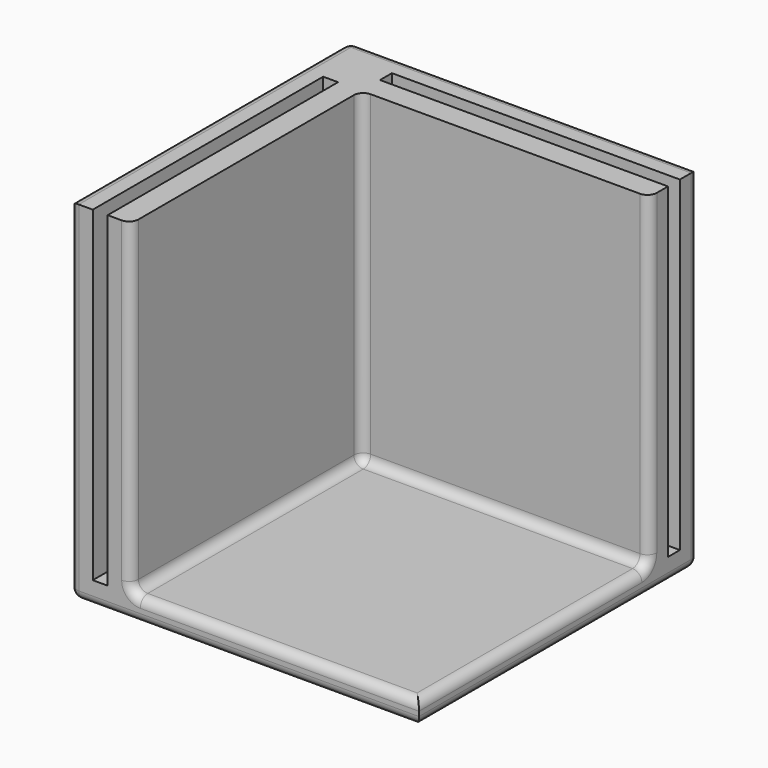
from build123d import *

# Parameters (mm, degrees)
F0_W     = 75
F0_H     = 75
F1_DEPTH = 5
F2_W     = 5
F2_H     = 5
F2_W_2   = 3.2
F2_H_2   = 3.2
F2_W_3   = 61.8
F2_H_3   = 61.8
F3_DEPTH = 70
F4_R     = 2
F5_W     = 3.2
F5_H     = 3.2
F6_DEPTH = 75


# Not quite as in the source:
# - a feature names something its author has since deleted; it is built from what else it names


with BuildPart() as f1:
    # F0 (on Top) → F1 (new body)
    with BuildSketch(Plane.XY):
        Rectangle(F0_W, F0_H)
    extrude(amount=F1_DEPTH)

    # F2 (on face) → F3 (join)
    with BuildSketch(Plane.XY.offset(5)):
        with Locations((-35, 35)):
            Rectangle(F2_W, F2_H)
        with Locations((-30.9, 35)):
            Rectangle(F2_W_2, F2_H)
        with Locations((-35, 30.9)):
            Rectangle(F2_W, F2_H_2)
        with Locations((-26.8, 35)):
            Rectangle(F2_W, F2_H)
        with Locations((-35, 26.8)):
            Rectangle(F2_W, F2_H)
        with Locations((-30.9, 26.8)):
            Rectangle(F2_W_2, F2_H)
        with Locations((-26.8, 30.9)):
            Rectangle(F2_W, F2_H_2)
        with Locations((6.6, 35)):
            Rectangle(F2_W_3, F2_H)
        with Locations((-35, -6.6)):
            Rectangle(F2_W, F2_H_3)
        with Locations((-26.8, 26.8)):
            Rectangle(F2_W, F2_H)
        with Locations((-26.8, -6.6)):
            Rectangle(F2_W, F2_H_3)
        with Locations((6.6, 26.8)):
            Rectangle(F2_W_3, F2_H)
    extrude(amount=F3_DEPTH)

    # F4
    f4_edges = [f1.edges().sort_by_distance(p)[0] for p in [
        (0, -37.5, 0),
        (37.5, 0, 0),
        (0, 37.5, 0),
        (-37.5, 0, 0),
        (-37.5, 37.5, 37.5),
        (-37.5, 0, 75),
        (-37.5, -37.5, 37.5),
        (37.5, 37.5, 37.5),
        (0, 37.5, 75),
        (-24.3, -6.6, 5),
        (6.6, 24.3, 5),
        (37.5, -6.6, 5),
        (6.6, -37.5, 5),
        (-24.3, 24.3, 40),
        (-24.3, -37.5, 40),
        (37.5, 24.3, 40),
    ]]
    fillet(f4_edges, radius=F4_R)

    # F5 (on face) → F6 (join, through all)
    with BuildSketch(Plane.XY.offset(75)):
        with Locations((-30.9, 30.9)):
            Rectangle(F5_W, F5_H)
    extrude(amount=-F6_DEPTH)


solid = f1.part
